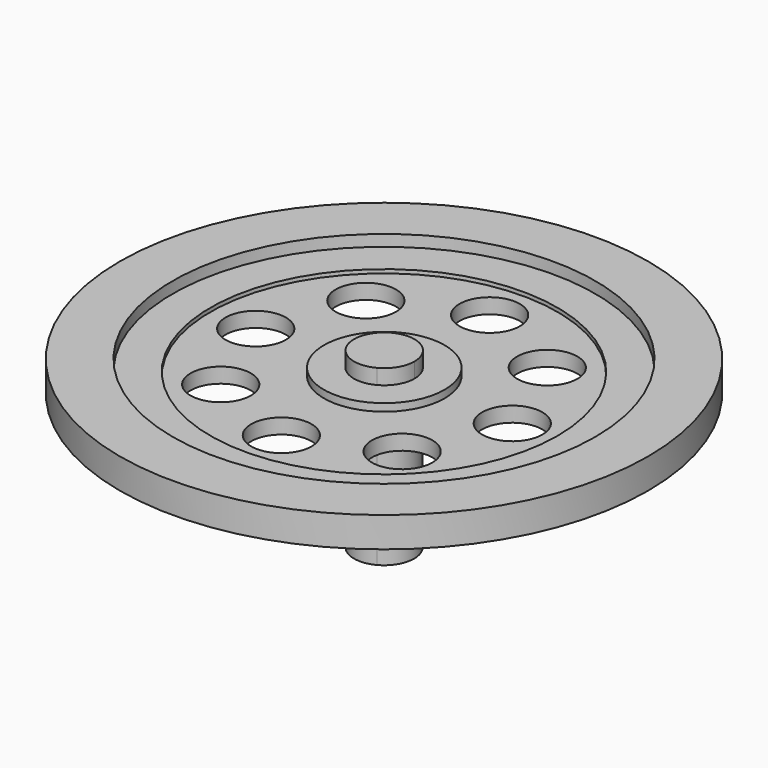
from build123d import *

# Parameters (mm, degrees)
F1_R      = 5.5
F1_R_2    = 2
F2_DEPTH  = 1
F1_R_3    = 11.5
F3_DEPTH  = 1
F1_R_4    = 14
F4_DEPTH  = 1.25
F1_R_5    = 17.5
F5_DEPTH  = 2
F7_DEPTH  = 1.5
F8_R      = 14.5
F8_R_2    = 11.5
F9_DEPTH  = 1
F10_DEPTH = 10
F11_R     = 1.325087
F12_DEPTH = 8
F13_R     = 4
F14_DEPTH = 0.5


with BuildPart() as f2:
    # F1 (on face) → F2 (new body)
    with BuildSketch(Plane.XY):
        with Locations((17.5, 17.5)):
            Circle(F1_R)
        with Locations((17.5, 17.5)):
            Circle(F1_R_2, mode=Mode.SUBTRACT)
    extrude(amount=F2_DEPTH)

    # F1 (on face) → F3 (join)
    with BuildSketch(Plane.XY):
        with Locations((17.5, 17.5)):
            Circle(F1_R_3)
        with Locations((11.489592, 11.489592)):
            Circle(F1_R_2, mode=Mode.SUBTRACT)
        with Locations((17.5, 9)):
            Circle(F1_R_2, mode=Mode.SUBTRACT)
        with Locations((23.510408, 11.489592)):
            Circle(F1_R_2, mode=Mode.SUBTRACT)
        with Locations((9, 17.5)):
            Circle(F1_R_2, mode=Mode.SUBTRACT)
        with Locations((11.489592, 23.510408)):
            Circle(F1_R_2, mode=Mode.SUBTRACT)
        with Locations((17.5, 17.5)):
            Circle(F1_R, mode=Mode.SUBTRACT)
        with Locations((26, 17.5)):
            Circle(F1_R_2, mode=Mode.SUBTRACT)
        with Locations((23.510408, 23.510408)):
            Circle(F1_R_2, mode=Mode.SUBTRACT)
        with Locations((17.5, 26.25)):
            Circle(F1_R_2, mode=Mode.SUBTRACT)
    extrude(amount=F3_DEPTH)

    # F1 (on face) → F4 (join)
    with BuildSketch(Plane.XY):
        with Locations((17.5, 17.5)):
            Circle(F1_R_4)
        with Locations((17.5, 17.5)):
            Circle(F1_R_3, mode=Mode.SUBTRACT)
    extrude(amount=F4_DEPTH)

    # F1 (on face) → F5 (join)
    with BuildSketch(Plane.XY):
        with Locations((17.5, 17.5)):
            Circle(F1_R_5)
        with Locations((17.5, 17.5)):
            Circle(F1_R_4, mode=Mode.SUBTRACT)
    extrude(amount=F5_DEPTH)

    # F6 (on face) → F7 (join)
    with BuildSketch(Plane.XY.offset(1)):
        with BuildLine():
            ThreePointArc((19.5, 17.5), (18.198396, 19.374098), (15.987757, 18.808862))
            ThreePointArc((15.987757, 18.808862), (15.943121, 16.261729), (18.434959, 15.731992))
            ThreePointArc((18.434959, 15.731992), (19.213172, 16.467992), (19.5, 17.5))
        make_face()
        with BuildLine():
            ThreePointArc((18.434959, 15.731992), (19.222275, 16.469381), (19.512816, 17.508223))
            ThreePointArc((19.512816, 17.508223), (18.203513, 19.3869), (15.987757, 18.808862))
            ThreePointArc((15.987757, 18.808862), (18.198396, 19.374098), (19.5, 17.5))
            ThreePointArc((19.5, 17.5), (19.213172, 16.467992), (18.434959, 15.731992))
        make_face()
    extrude(amount=F7_DEPTH)

    # F8 (on face) → F9 (cut)
    with BuildSketch(Plane(origin=(0, 0, 0), x_dir=(1, 0, 0), z_dir=(0, 0, -1))):
        with Locations((17.5, -17.5)):
            Circle(F8_R)
        with Locations((17.5, -17.5)):
            Circle(F8_R_2, mode=Mode.SUBTRACT)
    extrude(amount=-F9_DEPTH, mode=Mode.SUBTRACT)

    # F10 (add): a face of the model
    f10_faces = [f2.faces().sort_by_distance(p)[0] for p in [
        (17.503943, 17.503136, 1),
    ]]
    extrude(f10_faces, amount=F10_DEPTH)

    # F11 (on face) → F12 (cut)
    with BuildSketch(Plane(origin=(0, 0, -9), x_dir=(1, 0, 0), z_dir=(0, 0, -1))):
        with Locations((17.5, -17.5)):
            Circle(F11_R)
    extrude(amount=-F12_DEPTH, mode=Mode.SUBTRACT)

    # F13 (on face) → F14 (join)
    with BuildSketch(Plane.XY.offset(1)):
        with Locations((17.510338, 17.508223)):
            Circle(F13_R)
        with BuildLine():
            ThreePointArc((18.434959, 15.731992), (15.934722, 16.255049), (15.987757, 18.808862))
            ThreePointArc((15.987757, 18.808862), (19.077556, 18.754716), (18.434959, 15.731992))
        make_face(mode=Mode.SUBTRACT)
    extrude(amount=F14_DEPTH)


solid = f2.part
